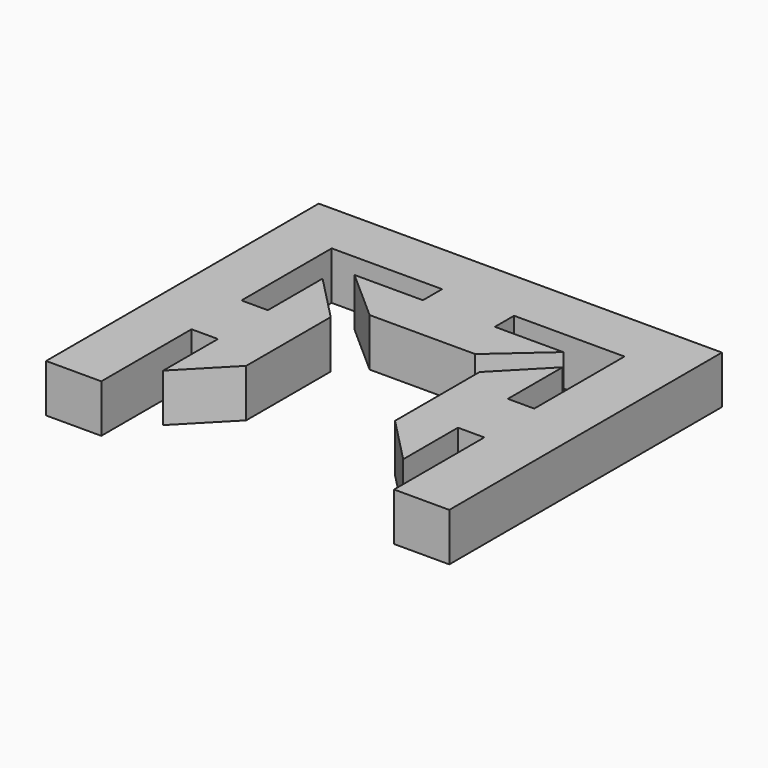
from build123d import *

# Parameters (mm, degrees)
F1_DEPTH = 5


# Not quite as in the source:
# - a feature names something its author has since deleted; it is built from what else it names


with BuildPart() as f1:
    # F0 (on Top) → F1 (new body)
    with BuildSketch(Plane.XY):
        Polygon((-3.25, -21), (-21, -21), (-21, -26.5), (-21, -56.5), (-15.25, -56.5), (-15.25, -44.75), (-15.25, -38.25), (-15.25, -26.5), (-3.75, -26.5), (0, -26.5), (3.75, -26.5), (15.25, -26.5), (15.25, -38.25), (15.25, -44.75), (15.25, -56.5), (21, -56.5), (21, -26.5), (21, -21), (3.25, -21), (0, -21), align=None)
        Polygon((0, -26.5), (-3.75, -26.5), (-3.75, -29), (-10.875, -29), (-5.5, -33.75), (0, -33.75), (5.5, -33.75), (10.875, -29), (3.75, -29), (3.75, -26.5), align=None)
        Polygon((-15.25, -38.25), (-15.25, -44.75), (-12.5, -44.75), (-12.5, -51.875), (-7.75, -47), (-7.75, -41.5), (-7.75, -36), (-12.5, -31.125), (-12.5, -38.25), align=None)
        Polygon((12.5, -44.75), (15.25, -44.75), (15.25, -38.25), (12.5, -38.25), (12.5, -31.125), (7.75, -36), (7.75, -41.5), (7.75, -47), (12.5, -51.875), align=None)
    extrude(amount=F1_DEPTH)


solid = f1.part
